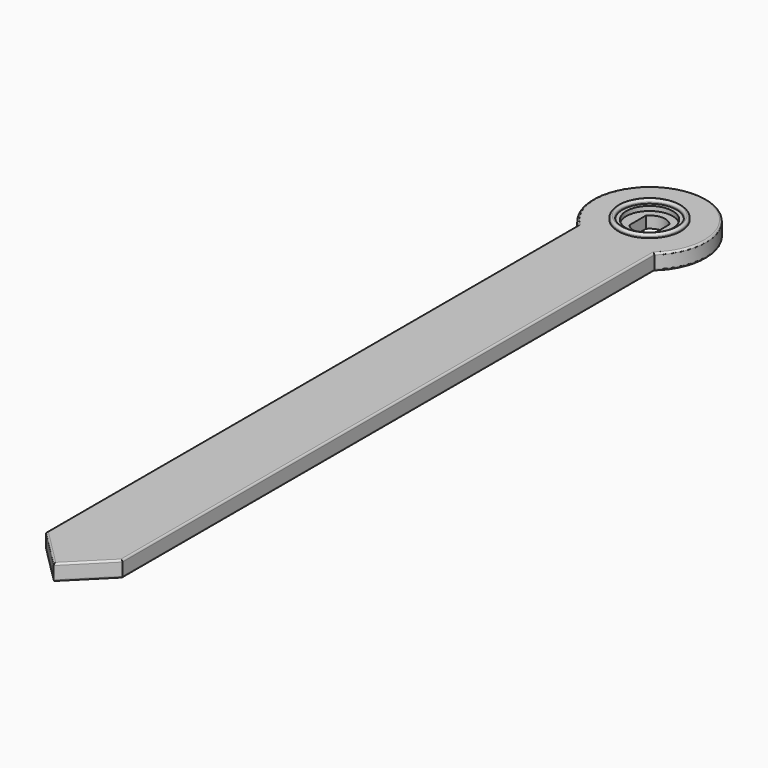
from build123d import *

# Parameters (mm, degrees)
F0_R     = 3.5
F0_R_2   = 3
F1_DEPTH = 1.8
F2_DEPTH = 2.2
F3_R     = 0.2
F4_R     = 0.24999
F5_R     = 2.5855494015
F6_DEPTH = 0.5


# Not quite as in the source:
# - a fillet or chamfer is up to 0.001 mm smaller than in the source, because OpenCascade refuses the exact size


with BuildPart() as f1:
    # F0 (on Top) → F1 (new body)
    with BuildSketch(Plane.XY):
        with BuildLine():
            Line((4.25, -78.75), (4.25, -4.6505376033))
            ThreePointArc((4.25, -4.6505376033), (0, 6.3), (-4.25, -4.6505376033))
            Line((-4.25, -4.6505376033), (-4.25, -78.75))
            Line((-4.25, -78.75), (0, -83))
            Line((0, -83), (4.25, -78.75))
        make_face()
        Circle(F0_R, mode=Mode.SUBTRACT)
        Circle(F0_R)
        Circle(F0_R_2, mode=Mode.SUBTRACT)
        Circle(F0_R_2)
        with BuildLine():
            ThreePointArc((1.325, -1.1431863365), (0, -1.75), (-1.325, -1.1431863365))
            Line((-1.325, -1.1431863365), (-1.325, 1.1431863365))
            ThreePointArc((-1.325, 1.1431863365), (0, 1.75), (1.325, 1.1431863365))
            Line((1.325, 1.1431863365), (1.325, -1.1431863365))
        make_face(mode=Mode.SUBTRACT)
    extrude(amount=F1_DEPTH)

    # F0 (on Top) → F2 (join)
    with BuildSketch(Plane.XY):
        Circle(F0_R)
        Circle(F0_R_2, mode=Mode.SUBTRACT)
    extrude(amount=F2_DEPTH)

    # F3
    f3_edges = [f1.edges().sort_by_distance(p)[0] for p in [
        (-4.25, -41.700269, 1.8),
        (0, 6.3, 1.8),
        (4.25, -41.700269, 1.8),
        (2.125, -80.875, 1.8),
        (-2.125, -80.875, 1.8),
        (0, 6.3, 0),
        (4.25, -41.700269, 0),
        (-4.25, -41.700269, 0),
        (-2.125, -80.875, 0),
        (2.125, -80.875, 0),
    ]]
    fillet(f3_edges, radius=F3_R)

    # F4 (radius 0.25 in the source; OpenCascade refuses exactly that, so slightly less here)
    f4_edges = [f1.edges().sort_by_distance(p)[0] for p in [
        (-3.5, 0, 2.2),
        (-3, 0, 2.2),
    ]]
    fillet(f4_edges, radius=F4_R)

    # F5 (on face) → F6 (cut)
    with BuildSketch(Plane.XY.offset(1.8)):
        Circle(F5_R)
    extrude(amount=-F6_DEPTH, mode=Mode.SUBTRACT)


solid = f1.part
